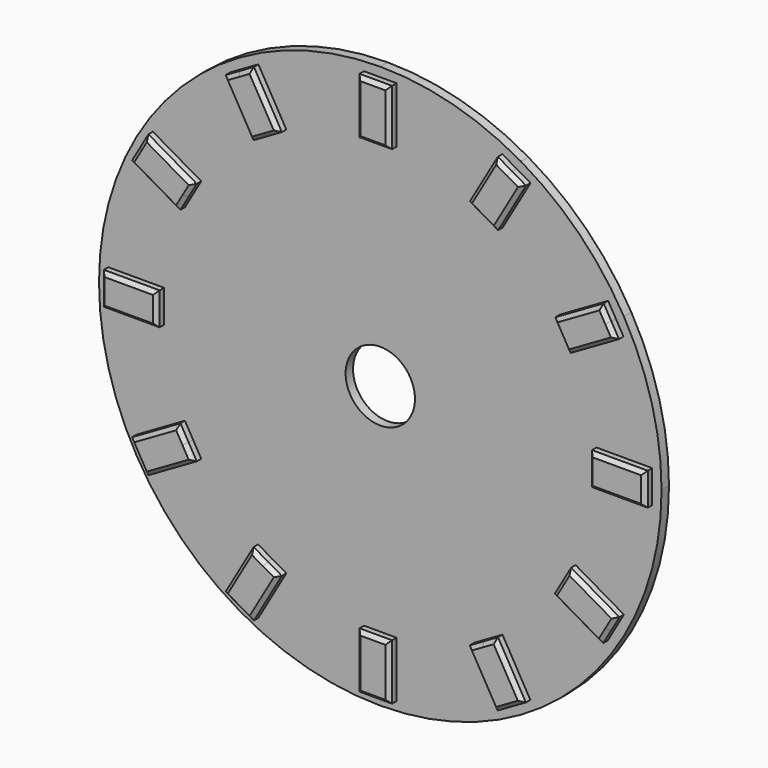
from build123d import *

# Parameters (mm, degrees)
F1_DEPTH   = 2
F0_W       = 12
F0_H       = 3.5
F2_DEPTH   = 2
F3_R       = 7.4577651792
F4_DEPTH   = 5
F6_DEPTH   = 2
F7_SIZE    = 0.8
F7_2_SIZE  = 0.8
F7_3_SIZE  = 0.8
F7_4_SIZE  = 0.8
F7_5_SIZE  = 0.8
F7_6_SIZE  = 0.8
F7_7_SIZE  = 0.8
F7_8_SIZE  = 0.8
F7_9_SIZE  = 0.8
F7_10_SIZE = 0.8
F7_11_SIZE = 0.8
F7_12_SIZE = 0.8


# Not quite as in the source:
# - the program builds the solid bodies; features that only make, move or delete a surface that nothing else refers to are left out


with BuildPart() as f1:
    # F0 (on Front) → F1 (new body)
    with BuildSketch(Plane.XZ):
        Polygon((-48.8832043045, 32.2641830484), (-50.6332043045, 29.2330941351), (-52.3832043045, 26.2020052219), (-41.9908994591, 20.2020052219), (-40.2408994591, 23.2330941351), (-38.4908994591, 26.2641830484), align=None)
    extrude(amount=F1_DEPTH)


with BuildPart() as f1b:
    # F0 (on Front) → F1, piece 2 (new body)
    with BuildSketch(Plane.XZ):
        Polygon((-26.2020052219, 52.3832043045), (-29.2330941351, 50.6332043045), (-32.2641830484, 48.8832043045), (-26.2641830484, 38.4908994591), (-23.2330941351, 40.2408994591), (-20.2020052219, 41.9908994591), align=None)
    extrude(amount=F1_DEPTH)


with BuildPart() as f1c:
    # F0 (on Front) → F1, piece 3 (new body)
    with BuildSketch(Plane.XZ):
        Polygon((3.5, 58.4661882703), (0, 58.4661882703), (-3.5, 58.4661882703), (-3.5, 46.4661882703), (0, 46.4661882703), (3.5, 46.4661882703), align=None)
    extrude(amount=F1_DEPTH)


with BuildPart() as f1d:
    # F0 (on Front) → F1, piece 4 (new body)
    with BuildSketch(Plane.XZ):
        Polygon((32.2973345277, 48.940624351), (29.2662456145, 50.690624351), (26.2351567012, 52.440624351), (20.2351567012, 42.0483195056), (23.2662456145, 40.2983195056), (26.2973345277, 38.5483195056), align=None)
    extrude(amount=F1_DEPTH)


with BuildPart() as f1e:
    # F0 (on Front) → F1, piece 5 (new body)
    with BuildSketch(Plane.XZ):
        Polygon((52.2771036984, 26.3857768623), (50.6332043045, 29.2330941351), (48.9893049106, 32.080411408), (38.5970000652, 26.080411408), (40.2408994591, 23.2330941351), (41.884798853, 20.3857768623), align=None)
    extrude(amount=F1_DEPTH)


with BuildPart() as f1f:
    # F0 (on Front) → F1, piece 6 (new body)
    with BuildSketch(Plane.XZ):
        Polygon((58.4661882703, -3.5), (58.4661882703, 0), (58.4661882703, 3.5), (46.4661882703, 3.5), (46.4661882703, 0), (46.4661882703, -3.5), align=None)
    extrude(amount=F1_DEPTH)


with BuildPart() as f1g:
    # F0 (on Front) → F1, piece 7 (new body)
    with BuildSketch(Plane.XZ):
        Polygon((48.8832043045, -32.2641830484), (50.6332043045, -29.2330941351), (52.3832043045, -26.2020052219), (41.9908994591, -20.2020052219), (40.2408994591, -23.2330941351), (38.4908994591, -26.2641830484), align=None)
    extrude(amount=F1_DEPTH)


with BuildPart() as f1h:
    # F0 (on Front) → F1, piece 8 (new body)
    with BuildSketch(Plane.XZ):
        Polygon((26.2020052219, -52.3832043045), (29.2330941351, -50.6332043045), (32.2641830484, -48.8832043045), (26.2641830484, -38.4908994591), (23.2330941351, -40.2408994591), (20.2020052219, -41.9908994591), align=None)
    extrude(amount=F1_DEPTH)


with BuildPart() as f1i:
    # F0 (on Front) → F1, piece 9 (new body)
    with BuildSketch(Plane.XZ):
        Polygon((-3.5, -58.4661882703), (0, -58.4661882703), (3.5, -58.4661882703), (3.5, -46.4661882703), (0, -46.4661882703), (-3.5, -46.4661882703), align=None)
    extrude(amount=F1_DEPTH)


with BuildPart() as f1j:
    # F0 (on Front) → F1, piece 10 (new body)
    with BuildSketch(Plane.XZ):
        Polygon((-32.2641830484, -48.8832043045), (-29.2330941351, -50.6332043045), (-26.2020052219, -52.3832043045), (-20.2020052219, -41.9908994591), (-23.2330941351, -40.2408994591), (-26.2641830484, -38.4908994591), align=None)
    extrude(amount=F1_DEPTH)


with BuildPart() as f1k:
    # F0 (on Front) → F1, piece 11 (new body)
    with BuildSketch(Plane.XZ):
        Polygon((-52.3832043045, -26.2020052219), (-50.6332043045, -29.2330941351), (-48.8832043045, -32.2641830484), (-38.4908994591, -26.2641830484), (-40.2408994591, -23.2330941351), (-41.9908994591, -20.2020052219), align=None)
    extrude(amount=F1_DEPTH)


with BuildPart() as f1l:
    # F0 (on Front) → F1, piece 12 (new body)
    with BuildSketch(Plane.XZ):
        with Locations((-52.4661882703, 1.75)):
            Rectangle(F0_W, F0_H)
        with Locations((-52.4661882703, -1.75)):
            Rectangle(F0_W, F0_H)
    extrude(amount=F1_DEPTH)


with BuildPart() as f2:
    # F0 (on Front) → F2 (new body)
    with BuildSketch(Plane.XZ):
        with BuildLine():
            Line((58.4661882703, 0), (60.4661882703, 0))
            ThreePointArc((60.4661882703, 0), (58.4058528675, 15.6498011091), (52.3652551121, 30.2330941351))
            Line((52.3652551121, 30.2330941351), (50.6332043045, 29.2330941351))
            Line((50.6332043045, 29.2330941351), (52.2771036984, 26.3857768623))
            Line((52.2771036984, 26.3857768623), (41.884798853, 20.3857768623))
            Line((41.884798853, 20.3857768623), (40.2408994591, 23.2330941351))
            Line((40.2408994591, 23.2330941351), (0, 0))
            Line((0, 0), (46.4661882703, 0))
            Line((46.4661882703, 0), (46.4661882703, 3.5))
            Line((46.4661882703, 3.5), (58.4661882703, 3.5))
            Line((58.4661882703, 3.5), (58.4661882703, 0))
        make_face()
        with BuildLine():
            ThreePointArc((52.3652551121, -30.2330941351), (58.4058528675, -15.6498011091), (60.4661882703, 0))
            Line((60.4661882703, 0), (58.4661882703, 0))
            Line((58.4661882703, 0), (58.4661882703, -3.5))
            Line((58.4661882703, -3.5), (46.4661882703, -3.5))
            Line((46.4661882703, -3.5), (46.4661882703, 0))
            Line((46.4661882703, 0), (0, 0))
            Line((0, 0), (40.2408994591, -23.2330941351))
            Line((40.2408994591, -23.2330941351), (41.9908994591, -20.2020052219))
            Line((41.9908994591, -20.2020052219), (52.3832043045, -26.2020052219))
            Line((52.3832043045, -26.2020052219), (50.6332043045, -29.2330941351))
            Line((50.6332043045, -29.2330941351), (52.3652551121, -30.2330941351))
        make_face()
        with BuildLine():
            Line((50.6332043045, 29.2330941351), (52.3652551121, 30.2330941351))
            ThreePointArc((52.3652551121, 30.2330941351), (42.7560517584, 42.7560517584), (30.2330941351, 52.3652551121))
            Line((30.2330941351, 52.3652551121), (29.2662456145, 50.690624351))
            Line((29.2662456145, 50.690624351), (32.2973345277, 48.940624351))
            Line((32.2973345277, 48.940624351), (26.2973345277, 38.5483195056))
            Line((26.2973345277, 38.5483195056), (23.2662456145, 40.2983195056))
            Line((23.2662456145, 40.2983195056), (0, 0))
            Line((0, 0), (40.2408994591, 23.2330941351))
            Line((40.2408994591, 23.2330941351), (38.5970000652, 26.080411408))
            Line((38.5970000652, 26.080411408), (48.9893049106, 32.080411408))
            Line((48.9893049106, 32.080411408), (50.6332043045, 29.2330941351))
        make_face()
        with BuildLine():
            ThreePointArc((30.2330941351, -52.3652551121), (42.7560517584, -42.7560517584), (52.3652551121, -30.2330941351))
            Line((52.3652551121, -30.2330941351), (50.6332043045, -29.2330941351))
            Line((50.6332043045, -29.2330941351), (48.8832043045, -32.2641830484))
            Line((48.8832043045, -32.2641830484), (38.4908994591, -26.2641830484))
            Line((38.4908994591, -26.2641830484), (40.2408994591, -23.2330941351))
            Line((40.2408994591, -23.2330941351), (0, 0))
            Line((0, 0), (23.2330941351, -40.2408994591))
            Line((23.2330941351, -40.2408994591), (26.2641830484, -38.4908994591))
            Line((26.2641830484, -38.4908994591), (32.2641830484, -48.8832043045))
            Line((32.2641830484, -48.8832043045), (29.2330941351, -50.6332043045))
            Line((29.2330941351, -50.6332043045), (30.2330941351, -52.3652551121))
        make_face()
        with BuildLine():
            Line((29.2662456145, 50.690624351), (30.2330941351, 52.3652551121))
            ThreePointArc((30.2330941351, 52.3652551121), (15.6498011091, 58.4058528675), (0, 60.4661882703))
            Line((0, 60.4661882703), (0, 58.4661882703))
            Line((0, 58.4661882703), (3.5, 58.4661882703))
            Line((3.5, 58.4661882703), (3.5, 46.4661882703))
            Line((3.5, 46.4661882703), (0, 46.4661882703))
            Line((0, 46.4661882703), (0, 0))
            Line((0, 0), (23.2662456145, 40.2983195056))
            Line((23.2662456145, 40.2983195056), (20.2351567012, 42.0483195056))
            Line((20.2351567012, 42.0483195056), (26.2351567012, 52.440624351))
            Line((26.2351567012, 52.440624351), (29.2662456145, 50.690624351))
        make_face()
        with BuildLine():
            ThreePointArc((0, -60.4661882703), (15.6498011091, -58.4058528675), (30.2330941351, -52.3652551121))
            Line((30.2330941351, -52.3652551121), (29.2330941351, -50.6332043045))
            Line((29.2330941351, -50.6332043045), (26.2020052219, -52.3832043045))
            Line((26.2020052219, -52.3832043045), (20.2020052219, -41.9908994591))
            Line((20.2020052219, -41.9908994591), (23.2330941351, -40.2408994591))
            Line((23.2330941351, -40.2408994591), (0, 0))
            Line((0, 0), (0, -46.4661882703))
            Line((0, -46.4661882703), (3.5, -46.4661882703))
            Line((3.5, -46.4661882703), (3.5, -58.4661882703))
            Line((3.5, -58.4661882703), (0, -58.4661882703))
            Line((0, -58.4661882703), (0, -60.4661882703))
        make_face()
        with BuildLine():
            Line((0, 58.4661882703), (0, 60.4661882703))
            ThreePointArc((0, 60.4661882703), (-15.6498011091, 58.4058528675), (-30.2330941351, 52.3652551121))
            Line((-30.2330941351, 52.3652551121), (-29.2330941351, 50.6332043045))
            Line((-29.2330941351, 50.6332043045), (-26.2020052219, 52.3832043045))
            Line((-26.2020052219, 52.3832043045), (-20.2020052219, 41.9908994591))
            Line((-20.2020052219, 41.9908994591), (-23.2330941351, 40.2408994591))
            Line((-23.2330941351, 40.2408994591), (0, 0))
            Line((0, 0), (0, 46.4661882703))
            Line((0, 46.4661882703), (-3.5, 46.4661882703))
            Line((-3.5, 46.4661882703), (-3.5, 58.4661882703))
            Line((-3.5, 58.4661882703), (0, 58.4661882703))
        make_face()
        with BuildLine():
            ThreePointArc((-30.2330941351, -52.3652551121), (-15.6498011091, -58.4058528675), (0, -60.4661882703))
            Line((0, -60.4661882703), (0, -58.4661882703))
            Line((0, -58.4661882703), (-3.5, -58.4661882703))
            Line((-3.5, -58.4661882703), (-3.5, -46.4661882703))
            Line((-3.5, -46.4661882703), (0, -46.4661882703))
            Line((0, -46.4661882703), (0, 0))
            Line((0, 0), (-23.2330941351, -40.2408994591))
            Line((-23.2330941351, -40.2408994591), (-20.2020052219, -41.9908994591))
            Line((-20.2020052219, -41.9908994591), (-26.2020052219, -52.3832043045))
            Line((-26.2020052219, -52.3832043045), (-29.2330941351, -50.6332043045))
            Line((-29.2330941351, -50.6332043045), (-30.2330941351, -52.3652551121))
        make_face()
        with BuildLine():
            Line((-29.2330941351, 50.6332043045), (-30.2330941351, 52.3652551121))
            ThreePointArc((-30.2330941351, 52.3652551121), (-42.7560517584, 42.7560517584), (-52.3652551121, 30.2330941351))
            Line((-52.3652551121, 30.2330941351), (-50.6332043045, 29.2330941351))
            Line((-50.6332043045, 29.2330941351), (-48.8832043045, 32.2641830484))
            Line((-48.8832043045, 32.2641830484), (-38.4908994591, 26.2641830484))
            Line((-38.4908994591, 26.2641830484), (-40.2408994591, 23.2330941351))
            Line((-40.2408994591, 23.2330941351), (0, 0))
            Line((0, 0), (-23.2330941351, 40.2408994591))
            Line((-23.2330941351, 40.2408994591), (-26.2641830484, 38.4908994591))
            Line((-26.2641830484, 38.4908994591), (-32.2641830484, 48.8832043045))
            Line((-32.2641830484, 48.8832043045), (-29.2330941351, 50.6332043045))
        make_face()
        with BuildLine():
            ThreePointArc((-52.3652551121, -30.2330941351), (-42.7560517584, -42.7560517584), (-30.2330941351, -52.3652551121))
            Line((-30.2330941351, -52.3652551121), (-29.2330941351, -50.6332043045))
            Line((-29.2330941351, -50.6332043045), (-32.2641830484, -48.8832043045))
            Line((-32.2641830484, -48.8832043045), (-26.2641830484, -38.4908994591))
            Line((-26.2641830484, -38.4908994591), (-23.2330941351, -40.2408994591))
            Line((-23.2330941351, -40.2408994591), (0, 0))
            Line((0, 0), (-40.2408994591, -23.2330941351))
            Line((-40.2408994591, -23.2330941351), (-38.4908994591, -26.2641830484))
            Line((-38.4908994591, -26.2641830484), (-48.8832043045, -32.2641830484))
            Line((-48.8832043045, -32.2641830484), (-50.6332043045, -29.2330941351))
            Line((-50.6332043045, -29.2330941351), (-52.3652551121, -30.2330941351))
        make_face()
        with BuildLine():
            Line((-50.6332043045, 29.2330941351), (-52.3652551121, 30.2330941351))
            ThreePointArc((-52.3652551121, 30.2330941351), (-58.4058528675, 15.6498011091), (-60.4661882703, 0))
            Line((-60.4661882703, 0), (-58.4661882703, 0))
            Line((-58.4661882703, 0), (-58.4661882703, 3.5))
            Line((-58.4661882703, 3.5), (-46.4661882703, 3.5))
            Line((-46.4661882703, 3.5), (-46.4661882703, 0))
            Line((-46.4661882703, 0), (0, 0))
            Line((0, 0), (-40.2408994591, 23.2330941351))
            Line((-40.2408994591, 23.2330941351), (-41.9908994591, 20.2020052219))
            Line((-41.9908994591, 20.2020052219), (-52.3832043045, 26.2020052219))
            Line((-52.3832043045, 26.2020052219), (-50.6332043045, 29.2330941351))
        make_face()
        with BuildLine():
            ThreePointArc((-60.4661882703, 0), (-58.4058528675, -15.6498011091), (-52.3652551121, -30.2330941351))
            Line((-52.3652551121, -30.2330941351), (-50.6332043045, -29.2330941351))
            Line((-50.6332043045, -29.2330941351), (-52.3832043045, -26.2020052219))
            Line((-52.3832043045, -26.2020052219), (-41.9908994591, -20.2020052219))
            Line((-41.9908994591, -20.2020052219), (-40.2408994591, -23.2330941351))
            Line((-40.2408994591, -23.2330941351), (0, 0))
            Line((0, 0), (-46.4661882703, 0))
            Line((-46.4661882703, 0), (-46.4661882703, -3.5))
            Line((-46.4661882703, -3.5), (-58.4661882703, -3.5))
            Line((-58.4661882703, -3.5), (-58.4661882703, 0))
            Line((-58.4661882703, 0), (-60.4661882703, 0))
        make_face()
    extrude(amount=-F2_DEPTH)

    # F3 (on Front) → F4 (cut)
    with BuildSketch(Plane.XZ):
        Circle(F3_R)
    extrude(amount=-F4_DEPTH, mode=Mode.SUBTRACT)


with BuildPart() as f6:
    # F6 (new): a face of the model
    f6_faces = [f1f.part.faces().sort_by_distance(p)[0] for p in [
        (52.4661882703, 0, 0),
    ]]
    extrude(f6_faces, amount=F6_DEPTH)


with BuildPart() as f6b:
    # F6#2 (new): a face of the model
    f6_2_faces = [f1e.part.faces().sort_by_distance(p)[0] for p in [
        (45.4370518818, 0, 26.2330941351),
    ]]
    extrude(f6_2_faces, amount=F6_DEPTH)


with BuildPart() as f6c:
    # F6#3 (new): a face of the model
    f6_3_faces = [f1d.part.faces().sort_by_distance(p)[0] for p in [
        (26.2662456145, 0, 45.4944719283),
    ]]
    extrude(f6_3_faces, amount=F6_DEPTH)


with BuildPart() as f6d:
    # F6#4 (new): a face of the model
    f6_4_faces = [f1c.part.faces().sort_by_distance(p)[0] for p in [
        (0, 0, 52.4661882703),
    ]]
    extrude(f6_4_faces, amount=F6_DEPTH)


with BuildPart() as f6e:
    # F6#5 (new): a face of the model
    f6_5_faces = [f1b.part.faces().sort_by_distance(p)[0] for p in [
        (-26.2330941351, 0, 45.4370518818),
    ]]
    extrude(f6_5_faces, amount=F6_DEPTH)


with BuildPart() as f6f:
    # F6#6 (new): a face of the model
    f6_6_faces = [f1.part.faces().sort_by_distance(p)[0] for p in [
        (-45.4370518818, 0, 26.2330941351),
    ]]
    extrude(f6_6_faces, amount=F6_DEPTH)


with BuildPart() as f6g:
    # F6#7 (new): a face of the model
    f6_7_faces = [f1l.part.faces().sort_by_distance(p)[0] for p in [
        (-52.4661882703, 0, 0),
    ]]
    extrude(f6_7_faces, amount=F6_DEPTH)


with BuildPart() as f6h:
    # F6#8 (new): a face of the model
    f6_8_faces = [f1k.part.faces().sort_by_distance(p)[0] for p in [
        (-45.4370518818, 0, -26.2330941351),
    ]]
    extrude(f6_8_faces, amount=F6_DEPTH)


with BuildPart() as f6i:
    # F6#9 (new): a face of the model
    f6_9_faces = [f1j.part.faces().sort_by_distance(p)[0] for p in [
        (-26.2330941351, 0, -45.4370518818),
    ]]
    extrude(f6_9_faces, amount=F6_DEPTH)


with BuildPart() as f6j:
    # F6#10 (new): a face of the model
    f6_10_faces = [f1i.part.faces().sort_by_distance(p)[0] for p in [
        (0, 0, -52.4661882703),
    ]]
    extrude(f6_10_faces, amount=F6_DEPTH)


with BuildPart() as f6k:
    # F6#11 (new): a face of the model
    f6_11_faces = [f1h.part.faces().sort_by_distance(p)[0] for p in [
        (26.2330941351, 0, -45.4370518818),
    ]]
    extrude(f6_11_faces, amount=F6_DEPTH)


with BuildPart() as f6l:
    # F6#12 (new): a face of the model
    f6_12_faces = [f1g.part.faces().sort_by_distance(p)[0] for p in [
        (45.4370518818, 0, -26.2330941351),
    ]]
    extrude(f6_12_faces, amount=F6_DEPTH)


with BuildPart() as f1_1:
    add(f1.part)

    # F7
    f7_edges = [f1_1.edges().sort_by_distance(p)[0] for p in [
        (-47.187052, -2, 23.202005),
        (-43.687052, -2, 29.264183),
        (-50.633204, -2, 29.233094),
        (-40.240899, -2, 23.233094),
    ]]
    chamfer(f7_edges, length=F7_SIZE)


with BuildPart() as f1b_1:
    add(f1b.part)

    # F7#2
    f7_2_edges = [f1b_1.edges().sort_by_distance(p)[0] for p in [
        (-29.264183, -2, 43.687052),
        (-23.202005, -2, 47.187052),
        (-29.233094, -2, 50.633204),
        (-23.233094, -2, 40.240899),
    ]]
    chamfer(f7_2_edges, length=F7_2_SIZE)


with BuildPart() as f1c_1:
    add(f1c.part)

    # F7#3
    f7_3_edges = [f1c_1.edges().sort_by_distance(p)[0] for p in [
        (-3.5, -2, 52.466188),
        (3.5, -2, 52.466188),
        (0, -2, 58.466188),
        (0, -2, 46.466188),
    ]]
    chamfer(f7_3_edges, length=F7_3_SIZE)


with BuildPart() as f1d_1:
    add(f1d.part)

    # F7#4
    f7_4_edges = [f1d_1.edges().sort_by_distance(p)[0] for p in [
        (23.235157, -2, 47.244472),
        (29.297335, -2, 43.744472),
        (29.266246, -2, 50.690624),
        (23.266246, -2, 40.29832),
    ]]
    chamfer(f7_4_edges, length=F7_4_SIZE)


with BuildPart() as f1e_1:
    add(f1e.part)

    # F7#5
    f7_5_edges = [f1e_1.edges().sort_by_distance(p)[0] for p in [
        (47.080951, -2, 23.385777),
        (43.793152, -2, 29.080411),
        (50.633204, -2, 29.233094),
        (40.240899, -2, 23.233094),
    ]]
    chamfer(f7_5_edges, length=F7_5_SIZE)


with BuildPart() as f1f_1:
    add(f1f.part)

    # F7#6
    f7_6_edges = [f1f_1.edges().sort_by_distance(p)[0] for p in [
        (52.466188, -2, -3.5),
        (58.466188, -2, 0),
        (52.466188, -2, 3.5),
        (46.466188, -2, 0),
    ]]
    chamfer(f7_6_edges, length=F7_6_SIZE)


with BuildPart() as f1g_1:
    add(f1g.part)

    # F7#7
    f7_7_edges = [f1g_1.edges().sort_by_distance(p)[0] for p in [
        (43.687052, -2, -29.264183),
        (50.633204, -2, -29.233094),
        (47.187052, -2, -23.202005),
        (40.240899, -2, -23.233094),
    ]]
    chamfer(f7_7_edges, length=F7_7_SIZE)


with BuildPart() as f1h_1:
    add(f1h.part)

    # F7#8
    f7_8_edges = [f1h_1.edges().sort_by_distance(p)[0] for p in [
        (23.202005, -2, -47.187052),
        (29.233094, -2, -50.633204),
        (29.264183, -2, -43.687052),
        (23.233094, -2, -40.240899),
    ]]
    chamfer(f7_8_edges, length=F7_8_SIZE)


with BuildPart() as f1i_1:
    add(f1i.part)

    # F7#9
    f7_9_edges = [f1i_1.edges().sort_by_distance(p)[0] for p in [
        (3.5, -2, -52.466188),
        (0, -2, -58.466188),
        (-3.5, -2, -52.466188),
        (0, -2, -46.466188),
    ]]
    chamfer(f7_9_edges, length=F7_9_SIZE)


with BuildPart() as f1j_1:
    add(f1j.part)

    # F7#10
    f7_10_edges = [f1j_1.edges().sort_by_distance(p)[0] for p in [
        (-23.233094, -2, -40.240899),
        (-23.202005, -2, -47.187052),
        (-29.233094, -2, -50.633204),
        (-29.264183, -2, -43.687052),
    ]]
    chamfer(f7_10_edges, length=F7_10_SIZE)


with BuildPart() as f1k_1:
    add(f1k.part)

    # F7#11
    f7_11_edges = [f1k_1.edges().sort_by_distance(p)[0] for p in [
        (-43.687052, -2, -29.264183),
        (-50.633204, -2, -29.233094),
        (-47.187052, -2, -23.202005),
        (-40.240899, -2, -23.233094),
    ]]
    chamfer(f7_11_edges, length=F7_11_SIZE)


with BuildPart() as f1l_1:
    add(f1l.part)

    # F7#12
    f7_12_edges = [f1l_1.edges().sort_by_distance(p)[0] for p in [
        (-52.466188, -2, 3.5),
        (-58.466188, -2, 0),
        (-52.466188, -2, -3.5),
        (-46.466188, -2, 0),
    ]]
    chamfer(f7_12_edges, length=F7_12_SIZE)


solid = Compound([f2.part, f6.part, f6b.part, f6c.part, f6d.part, f6e.part, f6f.part, f6g.part, f6h.part, f6i.part, f6j.part, f6k.part, f6l.part, f1_1.part, f1b_1.part, f1c_1.part, f1d_1.part, f1e_1.part, f1f_1.part, f1g_1.part, f1h_1.part, f1i_1.part, f1j_1.part, f1k_1.part, f1l_1.part])
